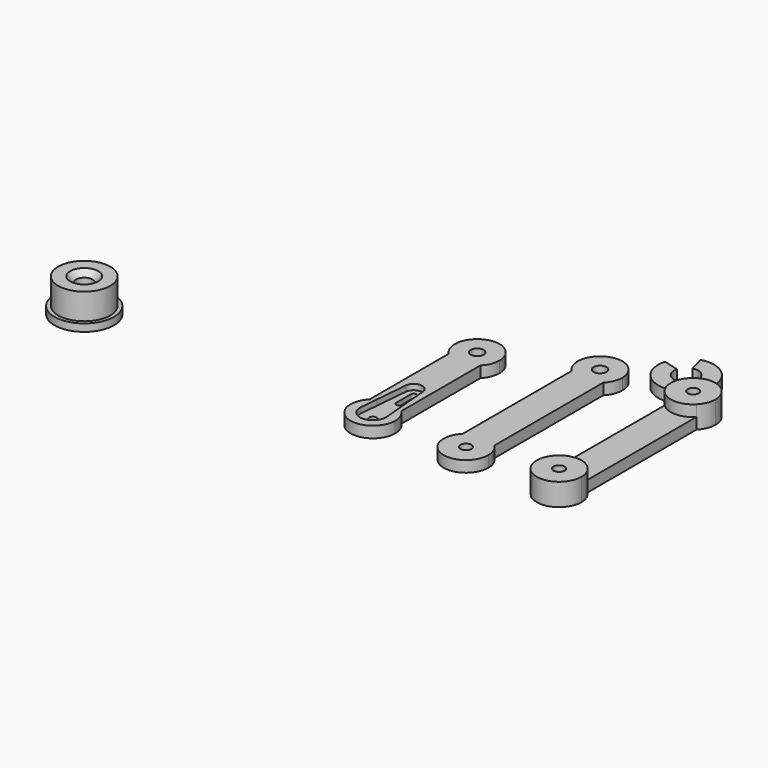
from build123d import *

# Parameters (mm, degrees)
F0_R     = 1.75
F0_R_2   = 1
F1_DEPTH = 3
F0_R_3   = 1.5
F2_DEPTH = 1.5
F3_DEPTH = 3
F0_R_4   = 8
F0_R_5   = 7
F0_R_6   = 3.3
F0_R_7   = 2.25
F4_DEPTH = 2
F5_DEPTH = 2
F6_DEPTH = 7
F7_W     = 5
F7_H     = 6
F8_DEPTH = 1.2
F9_SIZE  = 1.5


# Not quite as in the source:
# - a feature names something its author has since deleted; it is built from what else it names


with BuildPart() as f1:
    # F0 (on Top) → F1 (new body)
    with BuildSketch(Plane.XY):
        with BuildLine():
            ThreePointArc((3.059681, 5.161236), (3.684048, 4.735799), (4.25, 4.235269))
            Line((4.25, 4.235269), (4.25, 30.764731))
            ThreePointArc((4.25, 30.764731), (0, 29), (-4.25, 30.764731))
            Line((-4.25, 30.764731), (-4.25, 4.235269))
            ThreePointArc((-4.25, 4.235269), (-3.684048, 4.735799), (-3.059681, 5.161236))
            Line((-3.059681, 5.161236), (-2.29116, 13.90146))
            ThreePointArc((-2.29116, 13.90146), (0, 16), (2.29116, 13.90146))
            Line((2.29116, 13.90146), (3.059681, 5.161236))
        make_face()
        with BuildLine():
            ThreePointArc((-4.25, 30.764731), (0, 29), (4.25, 30.764731))
            ThreePointArc((4.25, 30.764731), (5.545268, 32.708712), (6, 35))
            ThreePointArc((6, 35), (-2.291288, 40.545268), (-4.25, 30.764731))
        make_face()
        with Locations((0, 35)):
            Circle(F0_R, mode=Mode.SUBTRACT)
        with BuildLine():
            ThreePointArc((2.3, 13.7), (2.297789, 13.800827), (2.29116, 13.90146))
            ThreePointArc((2.29116, 13.90146), (0, 16), (-2.29116, 13.90146))
            ThreePointArc((-2.29116, 13.90146), (-1.92956, 12.448281), (-0.75, 11.525719))
            Line((-0.75, 11.525719), (-0.75, 13.7))
            ThreePointArc((-0.75, 13.7), (0, 14.45), (0.75, 13.7))
            Line((0.75, 13.7), (0.75, 11.525719))
            ThreePointArc((0.75, 11.525719), (1.872832, 12.364897), (2.3, 13.7))
        make_face()
        with BuildLine():
            ThreePointArc((-3.059681, 5.161236), (0, 6), (3.059681, 5.161236))
            Line((3.059681, 5.161236), (2.29116, 13.90146))
            ThreePointArc((2.29116, 13.90146), (2.297789, 13.800827), (2.3, 13.7))
            ThreePointArc((2.3, 13.7), (1.872832, 12.364897), (0.75, 11.525719))
            Line((0.75, 11.525719), (0.75, 8.7))
            ThreePointArc((0.75, 8.7), (0, 7.95), (-0.75, 8.7))
            Line((-0.75, 8.7), (-0.75, 11.525719))
            ThreePointArc((-0.75, 11.525719), (-1.92956, 12.448281), (-2.29116, 13.90146))
            Line((-2.29116, 13.90146), (-3.059681, 5.161236))
        make_face()
        with BuildLine():
            Line((3.486548, 0.306569), (3.059681, 5.161236))
            ThreePointArc((3.059681, 5.161236), (0, 6), (-3.059681, 5.161236))
            Line((-3.059681, 5.161236), (-3.486548, 0.306569))
            ThreePointArc((-3.486548, 0.306569), (0, 3.5), (3.486548, 0.306569))
        make_face()
        with BuildLine():
            ThreePointArc((-4.25, 4.235269), (-2.291288, -5.545268), (6, 0))
            ThreePointArc((6, 0), (5.545268, 2.291288), (4.25, 4.235269))
            ThreePointArc((4.25, 4.235269), (3.684048, 4.735799), (3.059681, 5.161236))
            Line((3.059681, 5.161236), (3.486548, 0.306569))
            ThreePointArc((3.486548, 0.306569), (3.496635, 0.153432), (3.5, 0))
            ThreePointArc((3.5, 0), (-0.153432, -3.496635), (-3.486548, 0.306569))
            Line((-3.486548, 0.306569), (-3.059681, 5.161236))
            ThreePointArc((-3.059681, 5.161236), (-3.684048, 4.735799), (-4.25, 4.235269))
        make_face()
        with BuildLine():
            ThreePointArc((3.5, 0), (3.496635, 0.153432), (3.486548, 0.306569))
            ThreePointArc((3.486548, 0.306569), (0, 3.5), (-3.486548, 0.306569))
            ThreePointArc((-3.486548, 0.306569), (-0.153432, -3.496635), (3.5, 0))
        make_face()
        Circle(F0_R_2, mode=Mode.SUBTRACT)
    extrude(amount=-F1_DEPTH)

    # F0 (on Top) → F2 (cut)
    with BuildSketch(Plane.XY):
        with BuildLine():
            ThreePointArc((2.3, 13.7), (2.297789, 13.800827), (2.29116, 13.90146))
            ThreePointArc((2.29116, 13.90146), (0, 16), (-2.29116, 13.90146))
            ThreePointArc((-2.29116, 13.90146), (-1.92956, 12.448281), (-0.75, 11.525719))
            Line((-0.75, 11.525719), (-0.75, 13.7))
            ThreePointArc((-0.75, 13.7), (0, 14.45), (0.75, 13.7))
            Line((0.75, 13.7), (0.75, 11.525719))
            ThreePointArc((0.75, 11.525719), (1.872832, 12.364897), (2.3, 13.7))
        make_face()
        with BuildLine():
            ThreePointArc((-3.059681, 5.161236), (0, 6), (3.059681, 5.161236))
            Line((3.059681, 5.161236), (2.29116, 13.90146))
            ThreePointArc((2.29116, 13.90146), (2.297789, 13.800827), (2.3, 13.7))
            ThreePointArc((2.3, 13.7), (1.872832, 12.364897), (0.75, 11.525719))
            Line((0.75, 11.525719), (0.75, 8.7))
            ThreePointArc((0.75, 8.7), (0, 7.95), (-0.75, 8.7))
            Line((-0.75, 8.7), (-0.75, 11.525719))
            ThreePointArc((-0.75, 11.525719), (-1.92956, 12.448281), (-2.29116, 13.90146))
            Line((-2.29116, 13.90146), (-3.059681, 5.161236))
        make_face()
        with BuildLine():
            Line((3.486548, 0.306569), (3.059681, 5.161236))
            ThreePointArc((3.059681, 5.161236), (0, 6), (-3.059681, 5.161236))
            Line((-3.059681, 5.161236), (-3.486548, 0.306569))
            ThreePointArc((-3.486548, 0.306569), (0, 3.5), (3.486548, 0.306569))
        make_face()
        with BuildLine():
            ThreePointArc((3.5, 0), (3.496635, 0.153432), (3.486548, 0.306569))
            ThreePointArc((3.486548, 0.306569), (0, 3.5), (-3.486548, 0.306569))
            ThreePointArc((-3.486548, 0.306569), (-0.153432, -3.496635), (3.5, 0))
        make_face()
        Circle(F0_R_2, mode=Mode.SUBTRACT)
    extrude(amount=-F2_DEPTH, mode=Mode.SUBTRACT)


with BuildPart() as f1b:
    # F0 (on Top) → F1, piece 2 (new body)
    with BuildSketch(Plane.XY):
        with BuildLine():
            ThreePointArc((20.75, 40.764731), (25, 39), (29.25, 40.764731))
            ThreePointArc((29.25, 40.764731), (30.545268, 42.708712), (31, 45))
            ThreePointArc((31, 45), (22.708712, 50.545268), (20.75, 40.764731))
        make_face()
        with Locations((25, 45)):
            Circle(F0_R, mode=Mode.SUBTRACT)
        with BuildLine():
            ThreePointArc((20.75, 4.235269), (25, 6), (29.25, 4.235269))
            Line((29.25, 4.235269), (29.25, 40.764731))
            ThreePointArc((29.25, 40.764731), (25, 39), (20.75, 40.764731))
            Line((20.75, 40.764731), (20.75, 4.235269))
        make_face()
        with BuildLine():
            ThreePointArc((20.75, 4.235269), (22.708712, -5.545268), (31, 0))
            ThreePointArc((31, 0), (30.545268, 2.291288), (29.25, 4.235269))
            ThreePointArc((29.25, 4.235269), (25, 6), (20.75, 4.235269))
        make_face()
        with Locations((25, 0)):
            Circle(F0_R_3, mode=Mode.SUBTRACT)
    extrude(amount=-F1_DEPTH)


with BuildPart() as f1c:
    # F0 (on Top) → F1, piece 3 (new body)
    with BuildSketch(Plane.XY):
        with BuildLine():
            ThreePointArc((45.75, 40.764731), (50, 39), (54.25, 40.764731))
            ThreePointArc((54.25, 40.764731), (55.545268, 42.708712), (56, 45))
            ThreePointArc((56, 45), (54.246322, 49.238956), (50.010417, 50.999991))
            ThreePointArc((50.010417, 50.999991), (48.378974, 50.776874), (46.869621, 50.118665))
            ThreePointArc((46.869621, 50.118665), (45.969491, 49.030509), (44.881335, 48.130379))
            ThreePointArc((44.881335, 48.130379), (44.223126, 46.621026), (44.000009, 44.989583))
            ThreePointArc((44.000009, 44.989583), (44.456723, 42.703899), (45.75, 40.764731))
        make_face()
        with Locations((50, 45)):
            Circle(F0_R_3, mode=Mode.SUBTRACT)
        with BuildLine():
            Line((42.030626, 46.958966), (44.000009, 44.989583))
            ThreePointArc((44.000009, 44.989583), (44.223126, 46.621026), (44.881335, 48.130379))
            ThreePointArc((44.881335, 48.130379), (43.516801, 47.396662), (42.030626, 46.958966))
        make_face()
        with BuildLine():
            ThreePointArc((46.869621, 50.118665), (48.378974, 50.776874), (50.010417, 50.999991))
            Line((50.010417, 50.999991), (48.041034, 52.969374))
            ThreePointArc((48.041034, 52.969374), (47.603338, 51.483199), (46.869621, 50.118665))
        make_face()
        with BuildLine():
            ThreePointArc((46.869621, 50.118665), (45.757359, 49.242641), (44.881335, 48.130379))
            ThreePointArc((44.881335, 48.130379), (45.969491, 49.030509), (46.869621, 50.118665))
        make_face()
        with BuildLine():
            ThreePointArc((45.75, 4.235269), (50, 6), (54.25, 4.235269))
            Line((54.25, 4.235269), (54.25, 40.764731))
            ThreePointArc((54.25, 40.764731), (50, 39), (45.75, 40.764731))
            Line((45.75, 40.764731), (45.75, 4.235269))
        make_face()
        with BuildLine():
            ThreePointArc((45.75, 4.235269), (47.708712, -5.545268), (56, 0))
            ThreePointArc((56, 0), (55.545268, 2.291288), (54.25, 4.235269))
            ThreePointArc((54.25, 4.235269), (50, 6), (45.75, 4.235269))
        make_face()
        with Locations((50, 0)):
            Circle(F0_R_3, mode=Mode.SUBTRACT)
        with BuildLine():
            ThreePointArc((42.030626, 46.958966), (43.516801, 47.396662), (44.881335, 48.130379))
            ThreePointArc((44.881335, 48.130379), (45.757359, 49.242641), (46.869621, 50.118665))
            ThreePointArc((46.869621, 50.118665), (47.603338, 51.483199), (48.041034, 52.969374))
            ThreePointArc((48.041034, 52.969374), (48.134836, 53.648728), (48.16619, 54.33381))
            ThreePointArc((48.16619, 54.33381), (45.231901, 60.28396), (38.725048, 61.578253))
            Line((38.725048, 61.578253), (39.825029, 57.473068))
            ThreePointArc((39.825029, 57.473068), (42.644665, 56.912208), (43.91619, 54.33381))
            ThreePointArc((43.91619, 54.33381), (40.24198, 51.111614), (37.526932, 55.174971))
            Line((37.526932, 55.174971), (33.421747, 56.274952))
            ThreePointArc((33.421747, 56.274952), (35.157967, 49.243674), (42.030626, 46.958966))
        make_face()
    extrude(amount=-F1_DEPTH)

    # F0 (on Top) → F3 (join)
    with BuildSketch(Plane.XY):
        with BuildLine():
            ThreePointArc((45.75, 40.764731), (50, 39), (54.25, 40.764731))
            ThreePointArc((54.25, 40.764731), (55.545268, 42.708712), (56, 45))
            ThreePointArc((56, 45), (54.246322, 49.238956), (50.010417, 50.999991))
            ThreePointArc((50.010417, 50.999991), (48.378974, 50.776874), (46.869621, 50.118665))
            ThreePointArc((46.869621, 50.118665), (45.969491, 49.030509), (44.881335, 48.130379))
            ThreePointArc((44.881335, 48.130379), (44.223126, 46.621026), (44.000009, 44.989583))
            ThreePointArc((44.000009, 44.989583), (44.456723, 42.703899), (45.75, 40.764731))
        make_face()
        with Locations((50, 45)):
            Circle(F0_R_3, mode=Mode.SUBTRACT)
        with BuildLine():
            ThreePointArc((46.869621, 50.118665), (45.757359, 49.242641), (44.881335, 48.130379))
            ThreePointArc((44.881335, 48.130379), (45.969491, 49.030509), (46.869621, 50.118665))
        make_face()
        with BuildLine():
            ThreePointArc((45.75, 4.235269), (47.708712, -5.545268), (56, 0))
            ThreePointArc((56, 0), (55.545268, 2.291288), (54.25, 4.235269))
            ThreePointArc((54.25, 4.235269), (50, 6), (45.75, 4.235269))
        make_face()
        with Locations((50, 0)):
            Circle(F0_R_3, mode=Mode.SUBTRACT)
    extrude(amount=F3_DEPTH)


with BuildPart() as f4:
    # F0 (on Top) → F4 (new body)
    with BuildSketch(Plane.XY):
        with Locations((-77.517884, 0)):
            Circle(F0_R_4)
        with Locations((-77.517884, 0)):
            Circle(F0_R_5, mode=Mode.SUBTRACT)
        with Locations((-77.517884, 0)):
            Circle(F0_R_5)
        with Locations((-77.517884, 0)):
            Circle(F0_R_6, mode=Mode.SUBTRACT)
        with Locations((-77.517884, 0)):
            Circle(F0_R_6)
        with Locations((-77.517884, 0)):
            Circle(F0_R_7, mode=Mode.SUBTRACT)
        with Locations((-77.517884, 0)):
            Circle(F0_R_7)
    extrude(amount=-F4_DEPTH)

    # F0 (on Top) → F5 (join)
    with BuildSketch(Plane.XY):
        with Locations((-77.517884, 0)):
            Circle(F0_R_7)
    extrude(amount=F5_DEPTH)

    # F0 (on Top) → F6 (join)
    with BuildSketch(Plane.XY):
        with Locations((-77.517884, 0)):
            Circle(F0_R_5)
        with Locations((-77.517884, 0)):
            Circle(F0_R_6, mode=Mode.SUBTRACT)
        with Locations((-77.517884, 0)):
            Circle(F0_R_6)
        with Locations((-77.517884, 0)):
            Circle(F0_R_7, mode=Mode.SUBTRACT)
    extrude(amount=F6_DEPTH)

    # F7 (on face) → F8 (cut, symmetric)
    with BuildSketch(Plane.XY):
        with Locations((-77.517884, 0)):
            Rectangle(F7_W, F7_H)
    extrude(amount=F8_DEPTH, both=True, mode=Mode.SUBTRACT)

    # F9
    f9_edges = [f4.edges().sort_by_distance(p)[0] for p in [
        (-79.767884, 0, 7),
    ]]
    chamfer(f9_edges, length=F9_SIZE)


solid = Compound([f1.part, f1b.part, f1c.part, f4.part])
